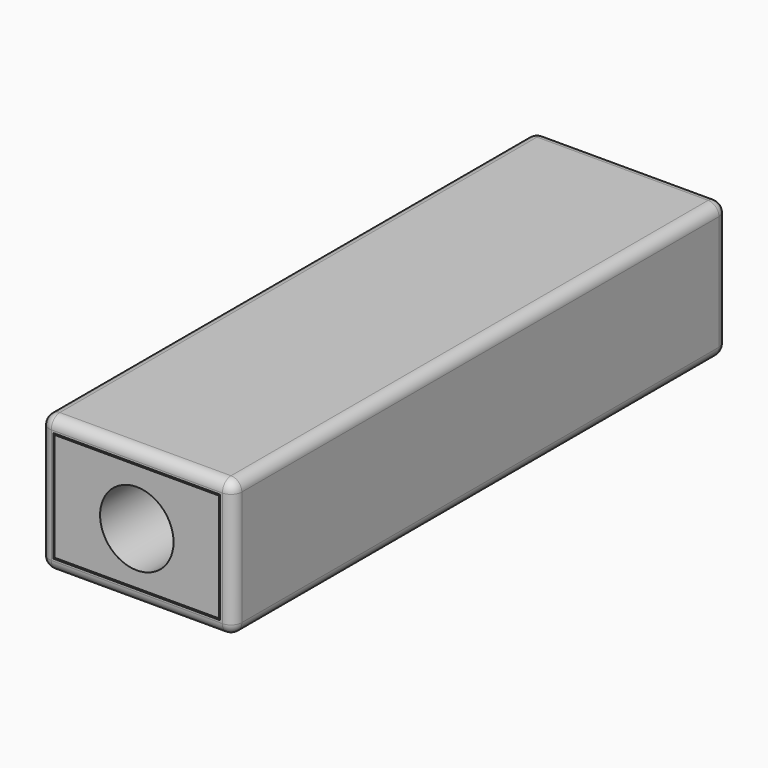
from build123d import *

# Parameters (mm, degrees)
F1_DEPTH = 3
F2_DEPTH = 25
F3_W     = 44.5999994099
F3_H     = 31.5999994099
F3_W_2   = 38.6
F3_H_2   = 25.6
F4_DEPTH = 140
F3_W_3   = 38
F3_H_3   = 25
F5_DEPTH = 3
F6_W     = 38
F6_H     = 25
F6_R     = 8.5
F7_DEPTH = 20
F6_R_2   = 3.5
F8_DEPTH = 7
F9_R     = 2.5


with BuildPart() as f1:
    # F0 (on Top) → F1 (new body)
    with BuildSketch(Plane.XY):
        Polygon((16, 110), (0, 110), (-16, 110), (-16, 50), (-16, 0), (0, 0), (16, 0), (16, 50), align=None)
    extrude(amount=F1_DEPTH)

    # F0 (on Top) → F2 (join)
    with BuildSketch(Plane.XY):
        Polygon((19, 113), (0, 113), (-19, 113), (-19, 47), (-19, -3), (-19, -7), (0, -7), (19, -7), (19, -3), (19, 47), align=None)
        Polygon((-16, 110), (0, 110), (16, 110), (16, 50), (16, 0), (0, 0), (-16, 0), (-16, 50), align=None, mode=Mode.SUBTRACT)
    extrude(amount=F2_DEPTH)

    # F6 (on face) → F7 (join)
    with BuildSketch(Plane.XZ.offset(7)):
        with Locations((0, 12.5)):
            Rectangle(F6_W, F6_H)
        with Locations((0, 12.1)):
            Circle(F6_R, mode=Mode.SUBTRACT)
    extrude(amount=F7_DEPTH)

    # F6 (on face) → F8 (cut, through all)
    with BuildSketch(Plane.XZ.offset(7)):
        with Locations((2.7, 15)):
            Circle(F6_R_2)
    extrude(amount=-F8_DEPTH, mode=Mode.SUBTRACT)


with BuildPart() as f4:
    # F3 (on face) → F4 (new body)
    with BuildSketch(Plane(origin=(0, 113, 0), x_dir=(-1, 0, 0), z_dir=(0, 1, 0))):
        with Locations((0, 12.5)):
            Rectangle(F3_W, F3_H)
        with Locations((0, 12.5)):
            Rectangle(F3_W_2, F3_H_2, mode=Mode.SUBTRACT)
    extrude(amount=-F4_DEPTH)

    # F3 (on face) → F5 (join)
    with BuildSketch(Plane(origin=(0, 113, 0), x_dir=(-1, 0, 0), z_dir=(0, 1, 0))):
        with Locations((0, 12.5)):
            Rectangle(F3_W, F3_H)
        with Locations((0, 12.5)):
            Rectangle(F3_W_2, F3_H_2, mode=Mode.SUBTRACT)
        with Locations((0, 12.5)):
            Rectangle(F3_W_2, F3_H_2)
        with Locations((0, 12.5)):
            Rectangle(F3_W_3, F3_H_3, mode=Mode.SUBTRACT)
        with Locations((0, 12.5)):
            Rectangle(F3_W_3, F3_H_3)
    extrude(amount=F5_DEPTH)

    # F9
    f9_edges = [f4.edges().sort_by_distance(p)[0] for p in [
        (0, 116, -3.3),
        (-22.3, 116, 12.5),
        (0, 116, 28.3),
        (22.3, 116, 12.5),
        (-22.3, 44.5, 28.3),
        (-22.3, 44.5, -3.3),
        (22.3, 44.5, -3.3),
        (22.3, 44.5, 28.3),
        (0, -27, -3.3),
        (22.3, -27, 12.5),
        (0, -27, 28.3),
        (-22.3, -27, 12.5),
    ]]
    fillet(f9_edges, radius=F9_R)


solid = Compound([f1.part, f4.part])
